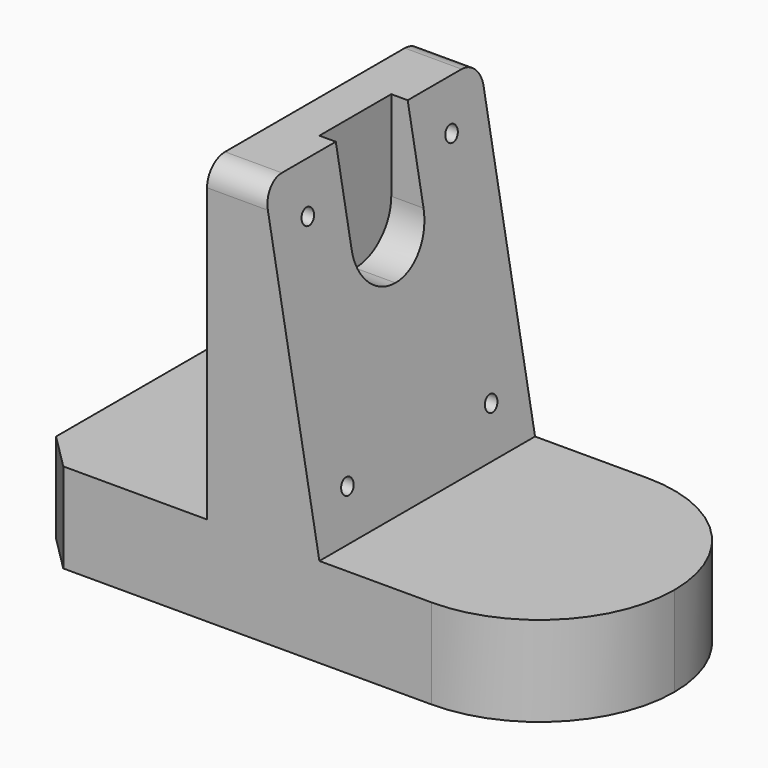
from build123d import *

# Parameters (mm, degrees)
F0_W           = 120
F0_H           = 60
F1_DEPTH       = 90
F2_W           = 40
F2_H           = 70
F2_W_2         = 55
F3_DEPTH       = 60.001
F4_R           = 29.99999
F5_SIZE        = 8
F7_D           = 3.4
F7_CBORE_D     = 7
F7_CBORE_DEPTH = 2.4
F9_DEPTH       = 16
F11_DEPTH      = 60.001
F12_R          = 5


# Not quite as in the source:
# - a fillet or chamfer is up to 0.001 mm smaller than in the source, because OpenCascade refuses the exact size


with BuildPart() as f1:
    # F0 (on Top) → F1 (new body)
    with BuildSketch(Plane.XY):
        Rectangle(F0_W, F0_H)
    extrude(amount=F1_DEPTH)

    # F2 (on face) → F3 (cut, through all)
    with BuildSketch(Plane.XZ.offset(30)):
        with Locations((-40, 55)):
            Rectangle(F2_W, F2_H)
        with Locations((32.5, 55)):
            Rectangle(F2_W_2, F2_H)
    extrude(amount=-F3_DEPTH, mode=Mode.SUBTRACT)

    # F4 (radius 30 in the source; OpenCascade refuses exactly that, so slightly less here)
    f4_edges = [f1.edges().sort_by_distance(p)[0] for p in [
        (60, -30, 10),
        (60, 30, 10),
    ]]
    fillet(f4_edges, radius=F4_R)

    # F5
    f5_edges = [f1.edges().sort_by_distance(p)[0] for p in [
        (-60, -30, 10),
        (-60, 30, 10),
    ]]
    chamfer(f5_edges, length=F5_SIZE)

    # F7 (through all)
    with Locations(Plane(origin=(-20, 0, 0), x_dir=(0, -1, 0), z_dir=(-1, 0, 0))):
        with Locations((-20, 80), (20, 80), (20, 30), (-20, 30)):
            CounterBoreHole(F7_D / 2, F7_CBORE_D / 2, F7_CBORE_DEPTH)

    # F8 (on face) → F9 (cut)
    with BuildSketch(Plane.YZ.offset(5)):
        with BuildLine():
            ThreePointArc((10, 70), (0, 80), (-10, 70))
            ThreePointArc((-10, 70), (-7.0710678119, 62.9289321881), (0, 60))
            ThreePointArc((0, 60), (7.0710678119, 62.9289321881), (10, 70))
        make_face()
        with BuildLine():
            Line((10, 90), (-10, 90))
            Line((-10, 90), (-10, 70))
            ThreePointArc((-10, 70), (0, 80), (10, 70))
            Line((10, 70), (10, 90))
        make_face()
    extrude(amount=-F9_DEPTH, mode=Mode.SUBTRACT)

    # F10 (on face) → F11 (cut, through all)
    with BuildSketch(Plane.XZ.offset(30)):
        Polygon((5, 90), (-7.3428886496, 90), (5, 20), align=None)
    extrude(amount=-F11_DEPTH, mode=Mode.SUBTRACT)

    # F12
    f12_edges = [f1.edges().sort_by_distance(p)[0] for p in [
        (-13.671444, -30, 90),
        (-13.671444, 30, 90),
    ]]
    fillet(f12_edges, radius=F12_R)


solid = f1.part
